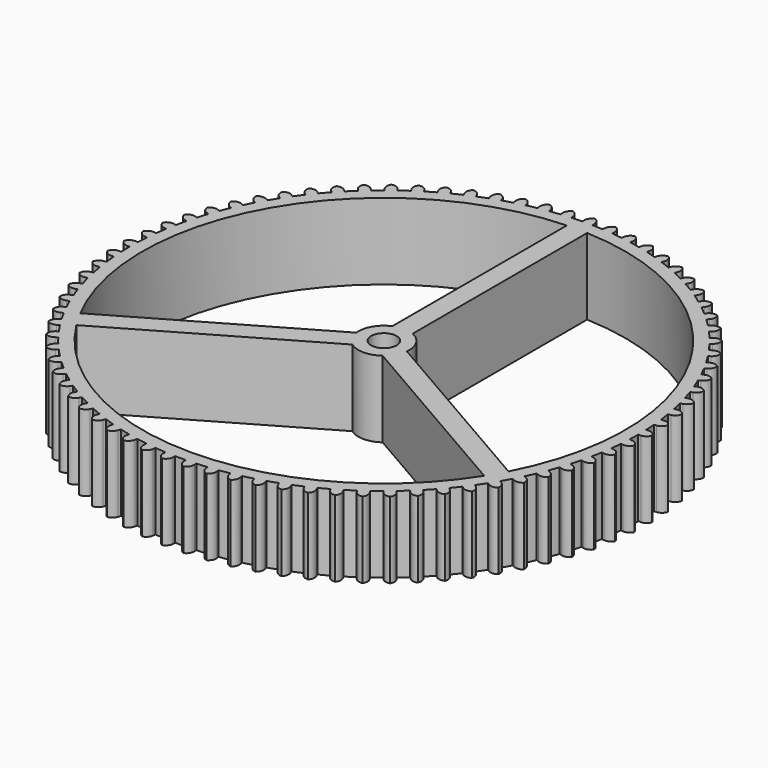
from build123d import *

# Parameters (mm, degrees)
F0_R        = 2.5
F1_DEPTH    = 15
F2_T1_DEPTH = 22.5


# Not quite as in the source:
# - a fillet or chamfer that OpenCascade refuses, or shapes differently, is made with other operations: its cross-section is extruded or revolved along the edge and cut away or added


with BuildPart() as f1:
    # F0 (on Top) → F1 (new body)
    with BuildSketch(Plane.XY):
        with BuildLine():
            Line((-1, 51.9899989998), (-1, 49.9899989998))
            ThreePointArc((-1, 49.9899989998), (-2.0393428715, 49.9583934955), (-3.0778037415, 49.9051813355))
            Line((-3.0778037415, 49.9051813355), (-3.2408225906, 51.8985299491))
            Line((-3.2408225906, 51.8985299491), (-5.2341677556, 51.735511382))
            Line((-5.2341677556, 51.735511382), (-5.0711491885, 49.742166217))
            Line((-5.0711491885, 49.742166217), (-7.1351257823, 49.4882704822))
            Line((-7.1351257823, 49.4882704822), (-7.460078617, 51.4616988431))
            Line((-7.460078617, 51.4616988431), (-9.4335035638, 51.1367465706))
            Line((-9.4335035638, 51.1367465706), (-9.1085512913, 49.1633216238))
            ThreePointArc((-9.1085512913, 49.1633216238), (-10.1289488194, 48.9632681136), (-11.1449653139, 48.7420374527))
            Line((-11.1449653139, 48.7420374527), (-11.6296896267, 50.6824127208))
            Line((-11.6296896267, 50.6824127208), (-13.5700615378, 50.1976892466))
            Line((-13.5700615378, 50.1976892466), (-13.0853380636, 48.2573173355))
            ThreePointArc((-13.0853380636, 48.2573173355), (-14.0860340848, 47.9747576153), (-15.0806375156, 47.6714483047))
            Line((-15.0806375156, 47.6714483047), (-15.7219075461, 49.5658576027))
            Line((-15.7219075461, 49.5658576027), (-17.6163135667, 48.9245886816))
            Line((-17.6163135667, 48.9245886816), (-16.9750446456, 47.030182661))
            ThreePointArc((-16.9750446456, 47.030182661), (-17.949379693, 46.6669971193), (-18.9159511383, 46.2836276323))
            Line((-18.9159511383, 46.2836276323), (-19.7094993403, 48.1194639789))
            Line((-19.7094993403, 48.1194639789), (-21.5453325108, 47.3259171498))
            Line((-21.5453325108, 47.3259171498), (-20.7517856817, 45.4900839793))
            ThreePointArc((-20.7517856817, 45.4900839793), (-21.6932757163, 45.0486895558), (-22.6253828026, 44.5878111532))
            Line((-22.6253828026, 44.5878111532), (-23.5659282438, 46.3528573604))
            Line((-23.5659282438, 46.3528573604), (-25.3309713973, 45.4123135464))
            Line((-25.3309713973, 45.4123135464), (-24.3904275833, 43.6472703928))
            ThreePointArc((-24.3904275833, 43.6472703928), (-25.2928071443, 43.1306044947), (-26.1842468528, 42.5952842462))
            Line((-26.1842468528, 42.5952842462), (-27.2655303584, 44.2777942227))
            Line((-27.2655303584, 44.2777942227), (-28.948037424, 43.1965125878))
            Line((-28.948037424, 43.1965125878), (-27.8667557891, 41.5140055221))
            ThreePointArc((-27.8667557891, 41.5140055221), (-28.7240196893, 40.9255064756), (-29.5688596358, 40.3193068491))
            Line((-29.5688596358, 40.3193068491), (-30.7836854425, 41.9080837686))
            Line((-30.7836854425, 41.9080837686), (-32.3724596133, 40.6932600636))
            Line((-32.3724596133, 40.6932600636), (-31.1576359083, 39.1044858928))
            ThreePointArc((-31.1576359083, 39.1044858928), (-31.964079198, 38.448070062), (-32.756697112, 37.775025216))
            Line((-32.756697112, 37.775025216), (-34.0969807544, 39.2594960302))
            Line((-34.0969807544, 39.2594960302), (-35.5814490004, 37.9192147066))
            Line((-35.5814490004, 37.9192147066), (-34.2411676768, 36.4347464606))
            ThreePointArc((-34.2411676768, 36.4347464606), (-34.9914236088, 35.7147821845), (-35.7265447489, 34.9793711214))
            Line((-35.7265447489, 34.9793711214), (-37.1833668606, 36.349656922))
            Line((-37.1833668606, 36.349656922), (-38.5536502905, 34.8928373307))
            Line((-38.5536502905, 34.8928373307), (-37.0968306992, 33.5225539008))
            ThreePointArc((-37.0968306992, 33.5225539008), (-37.7859064443, 32.743832423), (-38.4586387005, 31.9509491821))
            Line((-38.4586387005, 31.9509491821), (-40.0223043707, 33.1979309432))
            Line((-40.0223043707, 33.1979309432), (-41.2692839744, 31.6342679782))
            Line((-41.2692839744, 31.6342679782), (-39.7056210095, 30.3872883745))
            ThreePointArc((-39.7056210095, 30.3872883745), (-40.3289308821, 29.5549919579), (-40.9347973323, 28.7099130463))
            Line((-40.9347973323, 28.7099130463), (-42.5949006239, 29.82529231))
            Line((-42.5949006239, 29.82529231), (-43.7102779579, 28.1651918905))
            Line((-43.7102779579, 28.1651918905), (-42.0501775384, 27.0498145565))
            Line((-42.0501775384, 27.0498145565), (-43.1385422172, 25.2778312749))
            Line((-43.1385422172, 25.2778312749), (-44.8840354167, 26.2541853762))
            Line((-44.8840354167, 26.2541853762), (-45.8603878288, 24.5086951965))
            Line((-45.8603878288, 24.5086951965), (-44.1148976491, 23.5323427844))
            ThreePointArc((-44.1148976491, 23.5323427844), (-44.5946969692, 22.6098325488), (-45.0552077964, 21.6775438058))
            Line((-45.0552077964, 21.6775438058), (-46.8744749346, 22.5083752692))
            Line((-46.8744749346, 22.5083752692), (-47.7053049606, 20.6891112785))
            Line((-47.7053049606, 20.6891112785), (-45.8860409699, 19.8582812525))
            ThreePointArc((-45.8860409699, 19.8582812525), (-46.289050649, 18.8997324948), (-46.672038977, 17.9330099581))
            Line((-46.672038977, 17.9330099581), (-48.5529731311, 18.6127897373))
            Line((-48.5529731311, 18.6127897373), (-49.2327517343, 16.7318588373))
            Line((-49.2327517343, 16.7318588373), (-47.3518208343, 16.0520802341))
            ThreePointArc((-47.3518208343, 16.0520802341), (-47.6753589094, 15.0638719381), (-47.9782760139, 14.0691489867))
            Line((-47.9782760139, 14.0691489867), (-49.9083598777, 14.5933532595))
            Line((-49.9083598777, 14.5933532595), (-50.4325632435, 12.663272735))
            Line((-50.4325632435, 12.663272735), (-48.502482719, 12.1390693691))
            ThreePointArc((-48.502482719, 12.1390693691), (-48.7443960977, 11.127777898), (-48.9652261154, 10.1116742489))
            Line((-48.9652261154, 10.1116742489), (-50.931615299, 10.4768145223))
            Line((-50.931615299, 10.4768145223), (-51.2967549407, 8.5104287407))
            Line((-51.2967549407, 8.5104287407), (-49.3303691591, 8.1452890991))
            ThreePointArc((-49.3303691591, 8.1452890991), (-49.4890479477, 7.1176444307), (-49.6263212914, 6.0869220862))
            Line((-49.6263212914, 6.0869220862), (-51.6159297993, 6.2905684119))
            Line((-51.6159297993, 6.2905684119), (-51.8195757727, 4.3009633462))
            Line((-51.8195757727, 4.3009633462), (-49.8299707069, 4.0973173728))
            ThreePointArc((-49.8299707069, 4.0973173728), (-49.9043589243, 3.060158313), (-49.9571620624, 2.0216765601))
            Line((-49.9571620624, 2.0216765601), (-51.9567493782, 2.0624737055))
            Line((-51.9567493782, 2.0624737055), (-51.997546453, 0.0628898491))
            Line((-51.997546453, 0.0628898491), (-49.9979625966, 0.0220927743))
            ThreePointArc((-49.9979625966, 0.0220927743), (-49.9875652014, -1.0176785546), (-49.9555467378, -2.057008791))
            Line((-49.9555467378, -2.057008791), (-51.9518059378, -2.1793323243))
            Line((-51.9518059378, -2.1793323243), (-51.8294826162, -4.1755880707))
            Line((-51.8294826162, -4.1755880707), (-49.8332268698, -4.053264749))
            ThreePointArc((-49.8332268698, -4.053264749), (-49.738113055, -5.0887288404), (-49.6214860672, -6.1219909892))
            Line((-49.6214860672, -6.1219909892), (-51.6011323759, -6.4066211582))
            Line((-51.6011323759, -6.4066211582), (-51.3165026994, -8.3862640419))
            Line((-51.3165026994, -8.3862640419), (-49.3368598156, -8.1016343654))
            ThreePointArc((-49.3368598156, -8.1016343654), (-49.157662548, -9.1259003765), (-48.9572031694, -10.1462182485))
            Line((-48.9572031694, -10.1462182485), (-50.9070623672, -10.5912608864))
            Line((-50.9070623672, -10.5912608864), (-50.4620204993, -12.5411167107))
            Line((-50.4620204993, -12.5411167107), (-48.5121646749, -12.0960748428))
            ThreePointArc((-48.5121646749, -12.0960748428), (-48.2500764826, -13.1023264524), (-47.9671187374, -14.1029100005))
            Line((-47.9671187374, -14.1029100005), (-49.874214833, -14.705403422))
            Line((-49.874214833, -14.705403422), (-49.2717224539, -16.6124962181))
            Line((-49.2717224539, -16.6124962181), (-47.3646296577, -16.010003839))
            ThreePointArc((-47.3646296577, -16.010003839), (-47.0213946945, -16.9915446086), (-46.6578216197, -17.9657351144))
            Line((-46.6578216197, -17.9657351144), (-48.5094632032, -18.7216698251))
            Line((-48.5094632032, -18.7216698251), (-47.7535298004, -20.5733082052))
            Line((-47.7535298004, -20.5733082052), (-45.9018914203, -19.8173748023))
            ThreePointArc((-45.9018914203, -19.8173748023), (-45.4797938583, -20.76767274), (-45.0380249727, -21.7089871264))
            Line((-45.0380249727, -21.7089871264), (-46.8218896749, -22.6133325056))
            Line((-46.8218896749, -22.6133325056), (-45.9175458603, -24.3971941216))
            Line((-45.9175458603, -24.3971941216), (-44.1336842443, -23.492850307))
            ThreePointArc((-44.1336842443, -23.492850307), (-43.635533073, -24.4055813369), (-43.1185082758, -25.307755312))
            Line((-43.1185082758, -25.307755312), (-44.8227247714, -26.3544930903))
            Line((-44.8227247714, -26.3544930903), (-43.775988804, -28.0587066375))
            Line((-43.775988804, -28.0587066375), (-42.0717752568, -27.0119706701))
            ThreePointArc((-42.0717752568, -27.0119706701), (-41.5008855901, -27.8810607177), (-40.9120455958, -28.7380904625))
            Line((-40.9120455958, -28.7380904625), (-42.5252726053, -29.9202547728))
            Line((-42.5252726053, -29.9202547728), (-41.3431103402, -31.5334789913))
            Line((-41.3431103402, -31.5334789913), (-39.7298861218, -30.3513167262))
            ThreePointArc((-39.7298861218, -30.3513167262), (-39.0900571362, -31.1709821406), (-38.433320578, -31.9771642636))
            Line((-38.433320578, -31.9771642636), (-39.9448223417, -33.2868879974))
            Line((-39.9448223417, -33.2868879974), (-38.6351008738, -34.7983871461))
            Line((-38.6351008738, -34.7983871461), (-37.1236017251, -33.4886656782))
            ThreePointArc((-37.1236017251, -33.4886656782), (-36.419091377, -34.2534517214), (-35.6988287283, -35.0034212135))
            Line((-35.6988287283, -35.0034212135), (-37.0985464514, -36.4319883755))
            Line((-37.0985464514, -36.4319883755), (-35.6699817609, -37.831703677))
            Line((-35.6699817609, -37.831703677), (-34.2702664594, -36.4031389866))
            ThreePointArc((-34.2702664594, -36.4031389866), (-33.505763149, -37.1079561335), (-32.7267676388, -37.7967220716))
            Line((-32.7267676388, -37.7967220716), (-34.0053864308, -39.3346257829))
            Line((-34.0053864308, -39.3346257829), (-32.4674853801, -40.6132423628))
            Line((-32.4674853801, -40.6132423628), (-31.1888688002, -39.0753413121))
            ThreePointArc((-31.1888688002, -39.0753413121), (-30.3694601708, -39.7154991211), (-29.5369158858, -40.3384778814))
            Line((-29.5369158858, -40.3384778814), (-30.6859267495, -41.9754836467))
            Line((-30.6859267495, -41.9754836467), (-29.0489238163, -43.1244925225))
            Line((-29.0489238163, -43.1244925225), (-27.8999149405, -41.4874895894))
            ThreePointArc((-27.8999149405, -41.4874895894), (-27.0310540213, -42.0587279157), (-26.1505014063, -42.6117736774))
            Line((-26.1505014063, -42.6117736774), (-27.1622578641, -44.3369874933))
            Line((-27.1622578641, -44.3369874933), (-25.4370470329, -45.3487422007))
            Line((-25.4370470329, -45.3487422007), (-24.4252923255, -43.6235313695))
            ThreePointArc((-24.4252923255, -43.6235313695), (-23.5127612426, -44.1220487164), (-22.59006023, -44.6014810512))
            Line((-22.59006023, -44.6014810512), (-23.4578292095, -46.4034219044))
            Line((-23.4578292095, -46.4034219044), (-21.6558914737, -47.2711893827))
            Line((-21.6558914737, -47.2711893827), (-20.7881239955, -45.4692516469))
            ThreePointArc((-20.7881239955, -45.4692516469), (-19.8379954928, -45.8917304637), (-18.8792865055, -46.2943588284))
            Line((-18.8792865055, -46.2943588284), (-19.5972931474, -48.1610350999))
            Line((-19.5972931474, -48.1610350999), (-17.7306201053, -48.8790404996))
            Line((-17.7306201053, -48.8790404996), (-17.0126147056, -47.0123674576))
            ThreePointArc((-17.0126147056, -47.0123674576), (-16.0312117314, -47.3559962174), (-15.0428748197, -47.6791411868))
            Line((-15.0428748197, -47.6791411868), (-15.6063409082, -49.598130454))
            Line((-15.6063409082, -49.598130454), (-13.687354961, -50.1615955677))
            Line((-13.687354961, -50.1615955677), (-13.1238898473, -48.2426096204))
            ThreePointArc((-13.1238898473, -48.2426096204), (-12.1177434765, -48.5051015306), (-11.1063558594, -48.7466126282))
            Line((-11.1063558594, -48.7466126282), (-11.5115316207, -50.7051443341))
            Line((-11.5115316207, -50.7051443341), (-9.5530033032, -51.1103193944))
            Line((-9.5530033032, -51.1103193944), (-9.1478282429, -49.1517910769))
            ThreePointArc((-9.1478282429, -49.1517910769), (-8.1236342136, -49.3313992971), (-7.0959265088, -49.4896693063))
            Line((-7.0959265088, -49.4896693063), (-7.340115565, -51.4747097456))
            Line((-7.340115565, -51.4747097456), (-5.35507856, -51.7188983793))
            Line((-5.35507856, -51.7188983793), (-5.1108899263, -49.7338613743))
            ThreePointArc((-5.1108899263, -49.7338613743), (-4.0754640808, -49.8293906415), (-3.0382755136, -49.9033663016))
            Line((-3.0382755136, -49.9033663016), (-3.1198528268, -51.9017053575))
            Line((-3.1198528268, -51.9017053575), (-1.1215172281, -51.9832825297))
            Line((-1.1215172281, -51.9832825297), (-1.039940056, -49.984946931))
            ThreePointArc((-1.039940056, -49.984946931), (-0.0001729825, -49.9957615135), (1.0395941284, -49.9849505287))
            Line((1.0395941284, -49.9849505287), (1.1211714417, -51.9832895847))
            Line((1.1211714417, -51.9832895847), (3.1195070404, -51.9017124126))
            Line((3.1195070404, -51.9017124126), (3.0379298682, -49.9033768139))
            ThreePointArc((3.0379298682, -49.9033768139), (4.0751186914, -49.8294047425), (5.1105448674, -49.7338790582))
            Line((5.1105448674, -49.7338790582), (5.3547339237, -51.7189194974))
            Line((5.3547339237, -51.7189194974), (7.3397709286, -51.4747308636))
            Line((7.3397709286, -51.4747308636), (7.0955822949, -49.4896938587))
            ThreePointArc((7.0955822949, -49.4896938587), (8.1232905473, -49.3314274054), (9.147485198, -49.1518227291))
            Line((9.147485198, -49.1518227291), (9.5526609593, -51.110354435))
            Line((9.5526609593, -51.110354435), (11.5111892768, -50.7051793747))
            Line((11.5111892768, -50.7051793747), (11.1060142165, -48.7466510572))
            ThreePointArc((11.1060142165, -48.7466510572), (12.1174026693, -48.5051434592), (13.1235499484, -48.2426550304))
            Line((13.1235499484, -48.2426550304), (13.6870160369, -50.1616442976))
            Line((13.6870160369, -50.1616442976), (15.6060019841, -49.5981791839))
            Line((15.6060019841, -49.5981791839), (15.0425368704, -47.6791932367))
            ThreePointArc((15.0425368704, -47.6791932367), (16.0308749003, -47.3560516871), (17.0122790635, -47.0124263231))
            Line((17.0122790635, -47.0124263231), (17.7302857054, -48.8791025946))
            Line((17.7302857054, -48.8791025946), (19.5969587474, -48.1610971949))
            Line((19.5969587474, -48.1610971949), (18.8789533477, -46.2944241528))
            ThreePointArc((18.8789533477, -46.2944241528), (19.8376637281, -45.8917991054), (20.7877936927, -45.4693235762))
            Line((20.7877936927, -45.4693235762), (21.6555626722, -47.2712644295))
            Line((21.6555626722, -47.2712644295), (23.457500408, -46.4034969512))
            Line((23.457500408, -46.4034969512), (22.5897329298, -44.6015592154))
            ThreePointArc((22.5897329298, -44.6015592154), (23.5124356014, -44.1221300734), (24.4249684091, -43.6236158839))
            Line((24.4249684091, -43.6236158839), (25.4367248669, -45.3488296999))
            Line((25.4367248669, -45.3488296999), (27.1619356981, -44.3370749925))
            Line((27.1619356981, -44.3370749925), (26.1501809908, -42.6118641613))
            ThreePointArc((26.1501809908, -42.6118641613), (27.0307355194, -42.0588214465), (27.8995984151, -41.4875861265))
            Line((27.8995984151, -41.4875861265), (29.0486092789, -43.1245918918))
            Line((29.0486092789, -43.1245918918), (30.685612212, -41.9755830159))
            Line((30.685612212, -41.9755830159), (29.5366033361, -40.3385800828))
            ThreePointArc((29.5366033361, -40.3385800828), (30.3691497768, -39.7156042032), (31.1885606212, -39.0754492295))
            Line((31.1885606212, -39.0754492295), (32.4671794132, -40.6133529409))
            Line((32.4671794132, -40.6133529409), (34.0050804639, -39.334736361))
            Line((34.0050804639, -39.334736361), (32.726463884, -37.7968353103))
            ThreePointArc((32.726463884, -37.7968353103), (33.5054617774, -37.1080720677), (34.2699675266, -36.4032575661))
            Line((34.2699675266, -36.4032575661), (35.6696852497, -37.831824728))
            Line((35.6696852497, -37.831824728), (37.0982499402, -36.4321094265))
            Line((37.0982499402, -36.4321094265), (35.6985346387, -35.0035447361))
            ThreePointArc((35.6985346387, -35.0035447361), (36.4187998824, -34.2535777362), (37.1233128768, -33.4887941307))
            Line((37.1233128768, -33.4887941307), (38.6348146405, -34.7985178645))
            Line((38.6348146405, -34.7985178645), (39.9445361084, -33.2870187158))
            Line((39.9445361084, -33.2870187158), (38.4330369597, -31.9772972479))
            ThreePointArc((38.4330369597, -31.9772972479), (39.0897763074, -31.1711173973), (39.7296081291, -30.3514541968))
            Line((39.7296081291, -30.3514541968), (41.3428351386, -31.5336185071))
            Line((41.3428351386, -31.5336185071), (42.5249974036, -29.9203942886))
            Line((42.5249974036, -29.9203942886), (40.9117731851, -28.7382320236))
            ThreePointArc((40.9117731851, -28.7382320236), (41.5006161448, -27.8812043162), (42.0715088187, -27.012116244))
            Line((42.0715088187, -27.012116244), (43.7757253143, -28.0588540224))
            Line((43.7757253143, -28.0588540224), (44.8224612817, -26.3546404751))
            Line((44.8224612817, -26.3546404751), (43.1182477345, -25.3079045077))
            ThreePointArc((43.1182477345, -25.3079045077), (43.6352756534, -24.4057323216), (44.1334299829, -23.4930030154))
            Line((44.1334299829, -23.4930030154), (45.9172946851, -24.3973483946))
            Line((45.9172946851, -24.3973483946), (46.8216384997, -22.6134867786))
            Line((46.8216384997, -22.6134867786), (45.0377768837, -21.709142964))
            ThreePointArc((45.0377768837, -21.709142964), (45.4795490263, -20.7678301062), (45.9016498766, -19.817533629))
            Line((45.9016498766, -19.817533629), (47.7532914601, -20.5734683397))
            Line((47.7532914601, -20.5734683397), (48.5092248629, -18.7218299596))
            Line((48.5092248629, -18.7218299596), (46.6575864829, -17.9658965568))
            ThreePointArc((46.6575864829, -17.9658965568), (47.0211629285, -16.991707309), (47.364401288, -16.010167727))
            Line((47.364401288, -16.010167727), (49.2714973836, -16.6126611485))
            Line((49.2714973836, -16.6126611485), (49.8739897626, -14.7055683523))
            Line((49.8739897626, -14.7055683523), (47.9668969665, -14.1030759732))
            ThreePointArc((47.9668969665, -14.1030759732), (48.2498581739, -13.1024934042), (48.5119498479, -12.0962427015))
            Line((48.5119498479, -12.0962427015), (50.4618090457, -12.5412853394))
            Line((50.4618090457, -12.5412853394), (50.9068509136, -10.591429515))
            Line((50.9068509136, -10.591429515), (48.9569950892, -10.1463876471))
            ThreePointArc((48.9569950892, -10.1463876471), (49.1574579982, -9.1260704687), (49.33665881, -8.1018050776))
            Line((49.33665881, -8.1018050776), (51.3163051187, -8.3864352466))
            Line((51.3163051187, -8.3864352466), (51.6009347952, -6.4067923628))
            Line((51.6009347952, -6.4067923628), (49.6212919114, -6.1221626863))
            ThreePointArc((49.6212919114, -6.1221626863), (49.7379224744, -5.0889009411), (49.8330398721, -4.0534371788))
            Line((49.8330398721, -4.0534371788), (51.8292990721, -4.1757607121))
            Line((51.8292990721, -4.1757607121), (51.9516223938, -2.1795049657))
            Line((51.9516223938, -2.1795049657), (49.9553666474, -2.057181644))
            ThreePointArc((49.9553666474, -2.057181644), (49.9873887073, -1.0178515184), (49.9977897002, 0.0219197745))
            Line((49.9977897002, 0.0219197745), (51.997377016, 0.0627169199))
            Line((51.997377016, 0.0627169199), (51.9565799412, 2.0623007763))
            Line((51.9565799412, 2.0623007763), (49.9569960849, 2.0215037015))
            ThreePointArc((49.9569960849, 2.0215037015), (49.90419654, 3.059985637), (49.8298119114, 4.0971449543))
            Line((49.8298119114, 4.0971449543), (51.8194204193, 4.30079128))
            Line((51.8194204193, 4.30079128), (51.6157744459, 6.2903963457))
            Line((51.6157744459, 6.2903963457), (49.6261693802, 6.0867503723))
            ThreePointArc((49.6261693802, 6.0867503723), (49.4888996029, 7.1174731918), (49.3302243701, 8.1451184092))
            Line((49.3302243701, 8.1451184092), (51.2966135537, 8.5102586826))
            Line((51.2966135537, 8.5102586826), (50.9314739121, 10.4766444642))
            Line((50.9314739121, 10.4766444642), (48.9650881305, 10.1115048225))
            ThreePointArc((48.9650881305, 10.1115048225), (48.7442616285, 11.1276092356), (48.5023517491, 12.1389015438))
            Line((48.5023517491, 12.1389015438), (50.4324356128, 12.6631058166))
            Line((50.4324356128, 12.6631058166), (49.9082322469, 14.5931863411))
            Line((49.9082322469, 14.5931863411), (47.9781517224, 14.0689829752))
            ThreePointArc((47.9781517224, 14.0689829752), (47.6752380597, 15.0637069748), (47.3517034039, 16.0519163903))
            Line((47.3517034039, 16.0519163903), (49.2326375581, 16.7316961695))
            Line((49.2326375581, 16.7316961695), (48.5528589549, 18.6126270695))
            Line((48.5528589549, 18.6126270695), (46.6719280549, 17.9328484664))
            ThreePointArc((46.6719280549, 17.9328484664), (46.2889430719, 18.8995723283), (45.8859367096, 19.8581224804))
            Line((45.8859367096, 19.8581224804), (47.7052038477, 20.6889539438))
            Line((47.7052038477, 20.6889539438), (46.8743738217, 22.5082179345))
            Line((46.8743738217, 22.5082179345), (45.055109831, 21.6773879085))
            ThreePointArc((45.055109831, 21.6773879085), (44.5946022296, 22.609678245), (44.1148061015, 23.5321901407))
            Line((44.1148061015, 23.5321901407), (45.8602993011, 24.508544242))
            Line((45.8602993011, 24.508544242), (44.883946889, 26.2540344217))
            Line((44.883946889, 26.2540344217), (43.1384567093, 25.2776820096))
            ThreePointArc((43.1384567093, 25.2776820096), (42.6034910915, 26.1693345821), (42.0500981618, 27.049669057))
            Line((42.0500981618, 27.049669057), (43.7102014534, 28.1650483207))
            Line((43.7102014534, 28.1650483207), (42.5948241194, 29.8251487402))
            Line((42.5948241194, 29.8251487402), (40.9347236999, 28.7097714062))
            ThreePointArc((40.9347236999, 28.7097714062), (40.3288601738, 29.5548524142), (39.705553181, 30.3871509875))
            Line((39.705553181, 30.3871509875), (41.2692188512, 31.6341327486))
            Line((41.2692188512, 31.6341327486), (40.0222392475, 33.1977957135))
            Line((40.0222392475, 33.1977957135), (38.4585762826, 31.9508161098))
            ThreePointArc((38.4585762826, 31.9508161098), (37.7858467698, 32.7437016785), (37.0967737193, 33.5224255405))
            Line((37.0967737193, 33.5224255405), (38.553595831, 34.8927113412))
            Line((38.553595831, 34.8927113412), (37.1833124011, 36.3495309325))
            Line((37.1833124011, 36.3495309325), (35.7264928098, 34.9792475025))
            ThreePointArc((35.7264928098, 34.9792475025), (34.9913742143, 35.7146611093), (34.2411207735, 36.4346279813))
            Line((34.2411207735, 36.4346279813), (35.5814044159, 37.9190987955))
            Line((35.5814044159, 37.9190987955), (34.0969361699, 39.2593801192))
            Line((34.0969361699, 39.2593801192), (32.7566548462, 37.7749118732))
            ThreePointArc((32.7566548462, 37.7749118732), (31.9640392611, 38.4479594618), (31.1575982427, 39.104378083))
            Line((31.1575982427, 39.104378083), (32.3724240494, 40.6931550025))
            Line((32.3724240494, 40.6931550025), (30.7836498786, 41.9079787075))
            Line((30.7836498786, 41.9079787075), (29.5688261736, 40.3192045366))
            ThreePointArc((29.5688261736, 40.3192045366), (28.7239883247, 40.9254070865), (27.8667264608, 41.5139090992))
            Line((27.8667264608, 41.5139090992), (28.9480099664, 43.1964190757))
            Line((28.9480099664, 43.1964190757), (27.2655029008, 44.2777007106))
            Line((27.2655029008, 44.2777007106), (26.1842212658, 42.595193645))
            ThreePointArc((26.1842212658, 42.595193645), (25.2927834097, 43.130516978), (24.3904056365, 43.6471859985))
            Line((24.3904056365, 43.6471859985), (25.3309510776, 45.4122322057))
            Line((25.3309510776, 45.4122322057), (23.5659079241, 46.3527760197))
            Line((23.5659079241, 46.3527760197), (22.6253641101, 44.5877328661))
            ThreePointArc((22.6253641101, 44.5877328661), (21.6932586185, 45.048614494), (20.7517701112, 45.4900121752))
            Line((20.7517701112, 45.4900121752), (21.5453183132, 47.3258485218))
            Line((21.5453183132, 47.3258485218), (19.7094851427, 48.1193953509))
            Line((19.7094851427, 48.1193953509), (18.9159383136, 46.2835621804))
            ThreePointArc((18.9159383136, 46.2835621804), (17.9493681948, 46.6669350119), (16.9750344041, 47.030123925))
            Line((16.9750344041, 47.030123925), (17.6163044347, 48.924533223))
            Line((17.6163044347, 48.924533223), (15.7218984141, 49.5658021441))
            Line((15.7218984141, 49.5658021441), (15.080629493, 47.6713961235))
            ThreePointArc((15.080629493, 47.6713961235), (14.0860271117, 47.9747088756), (13.0853320682, 48.2572720584))
            Line((13.0853320682, 48.2572720584), (13.570056381, 50.1976473265))
            Line((13.570056381, 50.1976473265), (11.6296844699, 50.6823708007))
            Line((11.6296844699, 50.6823708007), (11.1449609957, 48.7419988895))
            ThreePointArc((11.1449609957, 48.7419988895), (10.1289452667, 48.963233066), (9.1085484308, 49.163290107))
            Line((9.1085484308, 49.163290107), (9.4335012655, 51.1367184679))
            Line((9.4335012655, 51.1367184679), (7.4600763188, 51.4616707404))
            Line((7.4600763188, 51.4616707404), (7.1351240462, 49.4882457936))
            ThreePointArc((7.1351240462, 49.4882457936), (6.1044563866, 49.6259291175), (5.0711483309, 49.7421486701))
            Line((5.0711483309, 49.7421486701), (5.23416718, 51.7354972838))
            Line((5.23416718, 51.7354972838), (3.2408220151, 51.8985158508))
            Line((3.2408220151, 51.8985158508), (3.077803448, 49.9051706859))
            ThreePointArc((3.077803448, 49.9051706859), (2.0393427808, 49.9583868973), (1, 49.9899955397))
            Line((1, 49.9899955397), (1, 51.9899989998))
            Line((1, 51.9899989998), (-1, 51.9899989998))
        make_face()
        with BuildLine():
            Line((-40.0997262765, -25.4609888369), (-2.9686269666, -4.023338655))
            ThreePointArc((-2.9686269666, -4.023338655), (0, -5), (2.9686269666, -4.023338655))
            Line((2.9686269666, -4.023338655), (40.0997262765, -25.4609888369))
            ThreePointArc((40.0997262765, -25.4609888369), (0, -47.5), (-40.0997262765, -25.4609888369))
        make_face(mode=Mode.SUBTRACT)
        Circle(F0_R, mode=Mode.SUBTRACT)
        with BuildLine():
            ThreePointArc((-42.0997262765, -21.9968872218), (-41.1362066798, 23.75), (-2, 47.4578760587))
            Line((-2, 47.4578760587), (-2, 4.582575695))
            ThreePointArc((-2, 4.582575695), (-4.3301270189, 2.5), (-4.9686269666, -0.5592370399))
            Line((-4.9686269666, -0.5592370399), (-42.0997262765, -21.9968872218))
        make_face(mode=Mode.SUBTRACT)
        with BuildLine():
            ThreePointArc((4.9686269666, -0.5592370399), (4.3301270189, 2.5), (2, 4.582575695))
            Line((2, 4.582575695), (2, 47.4578760587))
            ThreePointArc((2, 47.4578760587), (41.1362066798, 23.75), (42.0997262765, -21.9968872218))
            Line((42.0997262765, -21.9968872218), (4.9686269666, -0.5592370399))
        make_face(mode=Mode.SUBTRACT)
    extrude(amount=F1_DEPTH)

    # F2: fillet of radius 1.5 on 154 edges, made by hand

    # F2_s2 → F2_t1 (cut)
    with BuildSketch(Plane.XY.offset(-3.75)):
        with BuildLine():
            ThreePointArc((0.5, 51.9899989998), (-0.5606601718, 51.5506591716), (-1, 50.4899989998))
            Line((-1, 50.4899989998), (-1, 51.9899989998))
            Line((-1, 51.9899989998), (0.5, 51.9899989998))
        make_face()
        with BuildLine():
            ThreePointArc((1, 50.4899989998), (0.5606601718, 51.5506591716), (-0.5, 51.9899989998))
            Line((-0.5, 51.9899989998), (1, 51.9899989998))
            Line((1, 51.9899989998), (1, 50.4899989998))
        make_face()
        with BuildLine():
            ThreePointArc((4.7358308888, 51.7762519255), (3.6428897016, 51.424827615), (3.1185580897, 50.4035069771))
            Line((3.1185580897, 50.4035069771), (3.2408220151, 51.8985158508))
            Line((3.2408220151, 51.8985158508), (4.7358308888, 51.7762519255))
        make_face()
        with BuildLine():
            ThreePointArc((8.9401450289, 51.217956536), (7.8221961695, 50.9567864141), (7.2163621144, 49.9816020303))
            Line((7.2163621144, 49.9816020303), (7.4600763188, 51.4616707404))
            Line((7.4600763188, 51.4616707404), (8.9401450289, 51.217956536))
        make_face()
        with BuildLine():
            ThreePointArc((9.1897870612, 49.6566497578), (8.9286169392, 50.7745986171), (7.9534325555, 51.3804326723))
            Line((7.9534325555, 51.3804326723), (9.4335012655, 51.1367184679))
            Line((9.4335012655, 51.1367184679), (9.1897870612, 49.6566497578))
        make_face()
        with BuildLine():
            ThreePointArc((-3.1185586653, 50.4035210754), (-3.6428902771, 51.4248417133), (-4.7358314643, 51.7762660238))
            Line((-4.7358314643, 51.7762660238), (-3.2408225906, 51.8985299491))
            Line((-3.2408225906, 51.8985299491), (-3.1185586653, 50.4035210754))
        make_face()
        with BuildLine():
            ThreePointArc((-3.7391588818, 51.8577753073), (-4.7604795198, 51.3334436955), (-5.1119038302, 50.2405025083))
            Line((-5.1119038302, 50.2405025083), (-5.2341677556, 51.735511382))
            Line((-5.2341677556, 51.735511382), (-3.7391588818, 51.8577753073))
        make_face()
        with BuildLine():
            ThreePointArc((-7.2163644127, 49.9816301331), (-7.8221984678, 50.9568145168), (-8.9401473271, 51.2179846388))
            Line((-8.9401473271, 51.2179846388), (-7.460078617, 51.4616988431))
            Line((-7.460078617, 51.4616988431), (-7.2163644127, 49.9816301331))
        make_face()
        with BuildLine():
            ThreePointArc((-7.9534348537, 51.380460775), (-8.9286192375, 50.7746267199), (-9.1897893594, 49.6566778605))
            Line((-9.1897893594, 49.6566778605), (-9.4335035638, 51.1367465706))
            Line((-9.4335035638, 51.1367465706), (-7.9534348537, 51.380460775))
        make_face()
        with BuildLine():
            ThreePointArc((-11.266147021, 49.2271337875), (-11.9494517938, 50.1496922258), (-13.08496856, 50.3188701152))
            Line((-13.08496856, 50.3188701152), (-11.6296896267, 50.6824127208))
            Line((-11.6296896267, 50.6824127208), (-11.266147021, 49.2271337875))
        make_face()
        with BuildLine():
            ThreePointArc((-12.1147826045, 50.5612318523), (-13.0373410428, 49.8779270795), (-13.2065189322, 48.7424103133))
            Line((-13.2065189322, 48.7424103133), (-13.5700615378, 50.1976892466))
            Line((-13.5700615378, 50.1976892466), (-12.1147826045, 50.5612318523))
        make_face()
        with BuildLine():
            ThreePointArc((-15.2409558553, 48.1450530873), (-15.9971840651, 49.0088461061), (-17.1427120616, 49.0849059119))
            Line((-17.1427120616, 49.0849059119), (-15.7219075461, 49.5658576027))
            Line((-15.7219075461, 49.5658576027), (-15.2409558553, 48.1450530873))
        make_face()
        with BuildLine():
            ThreePointArc((-16.1955090513, 49.4055403725), (-17.0593020701, 48.6493121626), (-17.1353618759, 47.5037841662))
            Line((-17.1353618759, 47.5037841662), (-17.6163135667, 48.9245886816))
            Line((-17.6163135667, 48.9245886816), (-16.1955090513, 49.4055403725))
        make_face()
        with BuildLine():
            ThreePointArc((-19.1143392184, 46.7425891011), (-19.9384582914, 47.5418683003), (-21.0863742182, 47.5243038571))
            Line((-21.0863742182, 47.5243038571), (-19.7094993403, 48.1194639789))
            Line((-19.7094993403, 48.1194639789), (-19.1143392184, 46.7425891011))
        make_face()
        with BuildLine():
            ThreePointArc((-20.1684576329, 47.9210772717), (-20.9677368321, 47.0969581987), (-20.9501723889, 45.9490422719))
            Line((-20.9501723889, 45.9490422719), (-21.5453325108, 47.3259171498))
            Line((-21.5453325108, 47.3259171498), (-20.1684576329, 47.9210772717))
        make_face()
        with BuildLine():
            ThreePointArc((-22.8605203833, 45.0290749952), (-23.7470459429, 45.7585213036), (-24.8897106089, 45.6474494999))
            Line((-24.8897106089, 45.6474494999), (-23.5659282438, 46.3528573604))
            Line((-23.5659282438, 46.3528573604), (-22.8605203833, 45.0290749952))
        make_face()
        with BuildLine():
            ThreePointArc((-26.4545691322, 43.0159139234), (-27.3976014971, 43.6706729962), (-28.5274106576, 43.4668329965))
            Line((-28.5274106576, 43.4668329965), (-27.2655303584, 44.2777942227))
            Line((-27.2655303584, 44.2777942227), (-26.4545691322, 43.0159139234))
        make_face()
        with BuildLine():
            ThreePointArc((-27.6861571248, 44.0074738139), (-28.3409161976, 43.064441449), (-28.1370761978, 41.9346322885))
            Line((-28.1370761978, 41.9346322885), (-28.948037424, 43.1965125878))
            Line((-28.948037424, 43.1965125878), (-27.6861571248, 44.0074738139))
        make_face()
        with BuildLine():
            ThreePointArc((-24.0071890321, 46.1177214069), (-24.7366353405, 45.2311958473), (-24.6255635368, 44.0885311812))
            Line((-24.6255635368, 44.0885311812), (-25.3309713973, 45.4123135464))
            Line((-25.3309713973, 45.4123135464), (-24.0071890321, 46.1177214069))
        make_face()
        with BuildLine():
            ThreePointArc((-31.1808789852, 41.6043778423), (-31.7565935087, 40.6111143969), (-31.4613418346, 39.5016794355))
            Line((-31.4613418346, 39.5016794355), (-32.3724596133, 40.6932600636))
            Line((-32.3724596133, 40.6932600636), (-31.1808789852, 41.6043778423))
        make_face()
        with BuildLine():
            ThreePointArc((-29.8725676638, 40.7165031405), (-30.8658311092, 41.292217664), (-31.9752660706, 40.9969659899))
            Line((-31.9752660706, 40.9969659899), (-30.7836854425, 41.9080837686))
            Line((-30.7836854425, 41.9080837686), (-29.8725676638, 40.7165031405))
        make_face()
        with BuildLine():
            ThreePointArc((-33.0917697617, 38.1461448457), (-34.1286542833, 38.6389835349), (-35.2103319389, 38.2542850375))
            Line((-35.2103319389, 38.2542850375), (-34.0969807544, 39.2594960302))
            Line((-34.0969807544, 39.2594960302), (-33.0917697617, 38.1461448457))
        make_face()
        with BuildLine():
            ThreePointArc((-34.4680978159, 38.9244256993), (-34.9609365051, 37.8875411777), (-34.5762380077, 36.8058635221))
            Line((-34.5762380077, 36.8058635221), (-35.5814490004, 37.9192147066))
            Line((-35.5814490004, 37.9192147066), (-34.4680978159, 38.9244256993))
        make_face()
        with BuildLine():
            ThreePointArc((-36.0907521671, 35.3219443496), (-37.1643574695, 35.7286274442), (-38.2110794331, 35.2570422285))
            Line((-38.2110794331, 35.2570422285), (-37.1833668606, 36.349656922))
            Line((-37.1833668606, 36.349656922), (-36.0907521671, 35.3219443496))
        make_face()
        with BuildLine():
            ThreePointArc((-37.5259377181, 35.9854520242), (-37.9326208127, 34.9118467219), (-37.4610355971, 33.8651247583))
            Line((-37.4610355971, 33.8651247583), (-38.5536502905, 34.8928373307))
            Line((-38.5536502905, 34.8928373307), (-37.5259377181, 35.9854520242))
        make_face()
        with BuildLine():
            ThreePointArc((-38.849557147, 32.2626962404), (-39.9527385639, 32.5805173315), (-40.9575390735, 32.0251837195))
            Line((-40.9575390735, 32.0251837195), (-40.0223043707, 33.1979309432))
            Line((-40.0223043707, 33.1979309432), (-38.849557147, 32.2626962404))
        make_face()
        with BuildLine():
            ThreePointArc((-40.3340492716, 32.8070152019), (-40.6518703627, 31.703833785), (-40.0965367507, 30.6990332754))
            Line((-40.0965367507, 30.6990332754), (-41.2692839744, 31.6342679782))
            Line((-41.2692839744, 31.6342679782), (-40.3340492716, 32.8070152019))
        make_face()
        with BuildLine():
            ThreePointArc((-41.3498253093, 28.9887593095), (-42.4752413505, 29.2156033503), (-43.4314336244, 28.5802169954))
            Line((-43.4314336244, 28.5802169954), (-42.5949006239, 29.82529231))
            Line((-42.5949006239, 29.82529231), (-41.3498253093, 28.9887593095))
        make_face()
        with BuildLine():
            ThreePointArc((-42.8737449574, 29.4102672051), (-43.1005889982, 28.2848511639), (-42.4652026432, 27.32865889))
            Line((-42.4652026432, 27.32865889), (-43.7102779579, 28.1651918905))
            Line((-43.7102779579, 28.1651918905), (-42.8737449574, 29.4102672051))
        make_face()
        with BuildLine():
            ThreePointArc((-43.5749177819, 25.5219210671), (-44.7150789893, 25.6562784478), (-45.6162997257, 24.9450677414))
            Line((-45.6162997257, 24.9450677414), (-44.8840354167, 26.2541853762))
            Line((-44.8840354167, 26.2541853762), (-43.5749177819, 25.5219210671))
        make_face()
        with BuildLine():
            ThreePointArc((-45.1281235197, 25.8178128313), (-45.2624809004, 24.6776516239), (-44.551270194, 23.7764308874))
            Line((-44.551270194, 23.7764308874), (-45.8603878288, 24.5086951965))
            Line((-45.8603878288, 24.5086951965), (-45.1281235197, 25.8178128313))
        make_face()
        with BuildLine():
            ThreePointArc((-45.5100269416, 21.8852527497), (-46.6573457305, 21.9262293442), (-47.4975974541, 21.1439272762))
            Line((-47.4975974541, 21.1439272762), (-46.8744749346, 22.5083752692))
            Line((-46.8744749346, 22.5083752692), (-45.5100269416, 21.8852527497))
        make_face()
        with BuildLine():
            ThreePointArc((-47.0821824411, 22.0535592716), (-47.1231590356, 20.9062404827), (-46.3408569676, 20.065988759))
            Line((-46.3408569676, 20.065988759), (-47.7053049606, 20.6891112785))
            Line((-47.7053049606, 20.6891112785), (-47.0821824411, 22.0535592716))
        make_face()
        with BuildLine():
            ThreePointArc((-47.1422749561, 18.102955785), (-48.2891161092, 18.0502789007), (-49.0628070835, 17.2020915623))
            Line((-49.0628070835, 17.2020915623), (-48.5529731311, 18.6127897373))
            Line((-48.5529731311, 18.6127897373), (-47.1422749561, 18.102955785))
        make_face()
        with BuildLine():
            ThreePointArc((-48.7229177819, 18.1425570123), (-48.6702408977, 16.9957158592), (-47.8220535593, 16.2220248849))
            Line((-47.8220535593, 16.2220248849), (-49.2327517343, 16.7318588373))
            Line((-49.2327517343, 16.7318588373), (-48.7229177819, 18.1425570123))
        make_face()
        with BuildLine():
            ThreePointArc((-48.4607994843, 14.2002007351), (-49.599530963, 14.0542209281), (-50.3015124021, 13.1457928661))
            Line((-50.3015124021, 13.1457928661), (-49.9083598777, 14.5933532595))
            Line((-49.9083598777, 14.5933532595), (-48.4607994843, 14.2002007351))
        make_face()
        with BuildLine():
            ThreePointArc((-50.0394107191, 14.1108331284), (-49.8934309121, 12.9721016497), (-48.9850028501, 12.2701202106))
            Line((-48.9850028501, 12.2701202106), (-50.4325632435, 12.663272735))
            Line((-50.4325632435, 12.663272735), (-50.0394107191, 14.1108331284))
        make_face()
        with BuildLine():
            ThreePointArc((-49.4568259628, 10.2029597911), (-50.579869697, 9.9646485329), (-51.2054700303, 9.0020251861))
            Line((-51.2054700303, 9.0020251861), (-50.931615299, 10.4768145223))
            Line((-50.931615299, 10.4768145223), (-49.4568259628, 10.2029597911))
        make_face()
        with BuildLine():
            ThreePointArc((-51.0229002095, 9.9852180769), (-50.7845889512, 8.8621743428), (-49.8219656045, 8.2365740095))
            Line((-49.8219656045, 8.2365740095), (-51.2967549407, 8.5104287407))
            Line((-51.2967549407, 8.5104287407), (-51.0229002095, 9.9852180769))
        make_face()
        with BuildLine():
            ThreePointArc((-50.123726, 6.1378339319), (-51.2236083188, 5.8087771446), (-51.7686642793, 4.7983646127))
            Line((-51.7686642793, 4.7983646127), (-51.6159297993, 6.2905684119))
            Line((-51.6159297993, 6.2905684119), (-50.123726, 6.1378339319))
        make_face()
        with BuildLine():
            ThreePointArc((-51.6668412926, 5.7931671455), (-51.3377845053, 4.6932848266), (-50.3273719734, 4.1482288662))
            Line((-50.3273719734, 4.1482288662), (-51.8195757727, 4.3009633462))
            Line((-51.8195757727, 4.3009633462), (-51.6668412926, 5.7931671455))
        make_face()
        with BuildLine():
            ThreePointArc((-50.4570614859, 2.0318758994), (-51.5264628541, 1.6142634016), (-51.9873471843, 0.5627858132))
            Line((-51.9873471843, 0.5627858132), (-51.9567493782, 2.0624737055))
            Line((-51.9567493782, 2.0624737055), (-50.4570614859, 2.0318758994))
        make_face()
        with BuildLine():
            ThreePointArc((-51.9669486469, 1.5625777414), (-51.5493361491, 0.4931763732), (-50.4978585607, 0.032292043))
            Line((-50.4978585607, 0.032292043), (-51.997546453, 0.0628898491))
            Line((-51.997546453, 0.0628898491), (-51.9669486469, 1.5625777414))
        make_face()
        with BuildLine():
            ThreePointArc((-50.4546141281, -2.0875898331), (-51.4864178559, -2.5909788991), (-51.8600634466, -3.6765241341))
            Line((-51.8600634466, -3.6765241341), (-51.9518059378, -2.1793323243))
            Line((-51.9518059378, -2.1793323243), (-50.4546141281, -2.0875898331))
        make_face()
        with BuildLine():
            ThreePointArc((-51.9212251074, -2.6783962609), (-51.4178360414, -3.7101999888), (-50.3322908064, -4.0838455794))
            Line((-50.3322908064, -4.0838455794), (-51.8294826162, -4.1755880707))
            Line((-51.8294826162, -4.1755880707), (-51.9212251074, -2.6783962609))
        make_face()
        with BuildLine():
            ThreePointArc((-50.1164002131, -6.1931489008), (-51.1037398171, -6.7789645638), (-51.3876601185, -7.891353321))
            Line((-51.3876601185, -7.891353321), (-51.6011323759, -6.4066211582))
            Line((-51.6011323759, -6.4066211582), (-50.1164002131, -6.1931489008))
        make_face()
        with BuildLine():
            ThreePointArc((-51.5299749568, -6.9015318791), (-50.9441592937, -7.8888714831), (-49.8317705366, -8.1727917845))
            Line((-49.8317705366, -8.1727917845), (-51.3165026994, -8.3862640419))
            Line((-51.3165026994, -8.3862640419), (-51.5299749568, -6.9015318791))
        make_face()
        with BuildLine():
            ThreePointArc((-49.4446704989, -10.2574794854), (-50.3809753968, -10.9218232389), (-50.5732809662, -12.0536527547))
            Line((-50.5732809662, -12.0536527547), (-50.9070623672, -10.5912608864))
            Line((-50.9070623672, -10.5912608864), (-49.4446704989, -10.2574794854))
        make_face()
        with BuildLine():
            ThreePointArc((-50.7958019002, -11.0787248425), (-50.1314581467, -12.0150297404), (-48.999628631, -12.2073353098))
            Line((-48.999628631, -12.2073353098), (-50.4620204993, -12.5411167107))
            Line((-50.4620204993, -12.5411167107), (-50.7958019002, -11.0787248425))
        make_face()
        with BuildLine():
            ThreePointArc((-48.4438952358, -14.2535341377), (-49.3229344731, -14.9919848835), (-49.4223455487, -16.1357230191))
            Line((-49.4223455487, -16.1357230191), (-49.874214833, -14.705403422))
            Line((-49.874214833, -14.705403422), (-48.4438952358, -14.2535341377))
        make_face()
        with BuildLine():
            ThreePointArc((-49.7235917382, -15.182176621), (-48.9851409923, -16.0612158582), (-47.8414028568, -16.1606269338))
            Line((-47.8414028568, -16.1606269338), (-49.2717224539, -16.6124962181))
            Line((-49.2717224539, -16.6124962181), (-49.7235917382, -15.182176621))
        make_face()
        with BuildLine():
            ThreePointArc((-47.1207344182, -18.154719773), (-47.9366581336, -18.9623632434), (-47.9425131511, -20.1103986102))
            Line((-47.9425131511, -20.1103986102), (-48.5094632032, -18.7216698251))
            Line((-48.5094632032, -18.7216698251), (-47.1207344182, -18.154719773))
        make_face()
        with BuildLine():
            ThreePointArc((-48.3204798525, -19.1845794201), (-47.5128363821, -20.0005031356), (-46.3648010153, -20.006358153))
            Line((-46.3648010153, -20.006358153), (-47.7535298004, -20.5733082052))
            Line((-47.7535298004, -20.5733082052), (-48.3204798525, -19.1845794201))
        make_face()
        with BuildLine():
            ThreePointArc((-45.4839934629, -21.9350746447), (-46.2313718189, -22.8065361055), (-46.143631814, -23.9512287176))
            Line((-46.143631814, -23.9512287176), (-46.8218896749, -22.6133325056))
            Line((-46.8218896749, -22.6133325056), (-45.4839934629, -21.9350746447))
        make_face()
        with BuildLine():
            ThreePointArc((-46.5958037213, -23.0592979096), (-45.7243422604, -23.8066762656), (-44.5796496483, -23.7189362607))
            Line((-44.5796496483, -23.7189362607), (-45.9175458603, -24.3971941216))
            Line((-45.9175458603, -24.3971941216), (-46.5958037213, -23.0592979096))
        make_face()
        with BuildLine():
            ThreePointArc((-43.544564611, -25.5694411148), (-44.2184239278, -26.4989211338), (-44.0376727959, -27.6326532507))
            Line((-44.0376727959, -27.6326532507), (-44.8227247714, -26.3544930903))
            Line((-44.8227247714, -26.3544930903), (-43.544564611, -25.5694411148))
        make_face()
        with BuildLine():
            ThreePointArc((-44.5610407795, -26.7805464771), (-43.6315607605, -27.4544057939), (-42.4978286436, -27.273654662))
            Line((-42.4978286436, -27.273654662), (-43.775988804, -28.0587066375))
            Line((-43.775988804, -28.0587066375), (-44.5610407795, -26.7805464771))
        make_face()
        with BuildLine():
            ThreePointArc((-41.3153544414, -29.033633074), (-41.9112102965, -30.0149461151), (-41.6386509065, -31.1301729367))
            Line((-41.6386509065, -31.1301729367), (-42.5252726053, -29.9202547728))
            Line((-42.5252726053, -29.9202547728), (-41.3153544414, -29.033633074))
        make_face()
        with BuildLine():
            ThreePointArc((-42.229732039, -30.3235608274), (-41.2484189979, -30.9194166825), (-40.1331921764, -30.6468572925))
            Line((-40.1331921764, -30.6468572925), (-41.3431103402, -31.5334789913))
            Line((-41.3431103402, -31.5334789913), (-42.229732039, -30.3235608274))
        make_face()
        with BuildLine():
            ThreePointArc((-38.8111979802, -32.3045968965), (-39.3250850512, -33.3312124832), (-38.9625312408, -34.420512359))
            Line((-38.9625312408, -34.420512359), (-39.9448223417, -33.2868879974))
            Line((-39.9448223417, -33.2868879974), (-38.8111979802, -32.3045968965))
        make_face()
        with BuildLine():
            ThreePointArc((-39.6173919747, -33.6647627846), (-38.590776388, -34.1786498556), (-37.5014765123, -33.8160960452))
            Line((-37.5014765123, -33.8160960452), (-38.6351008738, -34.7983871461))
            Line((-38.6351008738, -34.7983871461), (-39.6173919747, -33.6647627846))
        make_face()
        with BuildLine():
            ThreePointArc((-36.0487599753, -35.3605648577), (-36.4772584285, -36.4256510327), (-36.0271229335, -37.4817748516))
            Line((-36.0271229335, -37.4817748516), (-37.0985464514, -36.4319883755))
            Line((-37.0985464514, -36.4319883755), (-36.0487599753, -35.3605648577))
        make_face()
        with BuildLine():
            ThreePointArc((-36.7414052788, -36.7819172009), (-35.6763191037, -37.2104156541), (-34.6201952848, -36.7602801592))
            Line((-34.6201952848, -36.7602801592), (-35.6699817609, -37.831703677))
            Line((-35.6699817609, -37.831703677), (-36.7414052788, -36.7819172009))
        make_face()
        with BuildLine():
            ThreePointArc((-33.0464239959, -38.1811999949), (-33.3866822448, -39.2776687855), (-32.8519606428, -40.2935882178))
            Line((-32.8519606428, -40.2935882178), (-34.0053864308, -39.3346257829))
            Line((-34.0053864308, -39.3346257829), (-33.0464239959, -38.1811999949))
        make_face()
        with BuildLine():
            ThreePointArc((-33.6209111681, -39.6542799279), (-32.5244423775, -39.9945381768), (-31.5085229452, -39.4598165748))
            Line((-31.5085229452, -39.4598165748), (-32.4674853801, -40.6132423628))
            Line((-32.4674853801, -40.6132423628), (-33.6209111681, -39.6542799279))
        make_face()
        with BuildLine():
            ThreePointArc((-29.8241700926, -40.7477314468), (-30.0739237747, -41.868286034), (-29.4581745496, -42.8372403036))
            Line((-29.4581745496, -42.8372403036), (-30.6859267495, -41.9754836467))
            Line((-30.6859267495, -41.9754836467), (-29.8241700926, -40.7477314468))
        make_face()
        with BuildLine():
            ThreePointArc((-30.2766760162, -42.2627358656), (-29.156121429, -42.5124895477), (-28.1871671594, -41.8967403227))
            Line((-28.1871671594, -41.8967403227), (-29.0489238163, -43.1244925225))
            Line((-29.0489238163, -43.1244925225), (-30.2766760162, -42.2627358656))
        make_face()
        with BuildLine():
            ThreePointArc((-26.4034418335, -43.0430793699), (-26.5610288793, -44.1802626479), (-25.8683497407, -45.0958035239))
            Line((-25.8683497407, -45.0958035239), (-27.1622578641, -44.3369874933))
            Line((-27.1622578641, -44.3369874933), (-26.4034418335, -43.0430793699))
        make_face()
        with BuildLine():
            ThreePointArc((-26.7309551563, -44.5899261702), (-25.5937718783, -44.7475132159), (-24.6782310023, -44.0548340773))
            Line((-24.6782310023, -44.0548340773), (-25.4370470329, -45.3487422007))
            Line((-25.4370470329, -45.3487422007), (-26.7309551563, -44.5899261702))
        make_face()
        with BuildLine():
            ThreePointArc((-22.8070036008, -45.0519686026), (-22.8713752945, -46.1982128042), (-22.1063759077, -47.0542475131))
            Line((-22.1063759077, -47.0542475131), (-23.4578292095, -46.4034219044))
            Line((-23.4578292095, -46.4034219044), (-22.8070036008, -45.0519686026))
        make_face()
        with BuildLine():
            ThreePointArc((-23.0073447756, -46.620363774), (-21.861100574, -46.6847354676), (-21.005065865, -45.9197360808))
            Line((-21.005065865, -45.9197360808), (-21.6558914737, -47.2711893827))
            Line((-21.6558914737, -47.2711893827), (-23.0073447756, -46.620363774))
        make_face()
        with BuildLine():
            ThreePointArc((-19.0587890976, -46.7610303184), (-19.0295170561, -47.9087073776), (-18.1972883658, -48.6995391497))
            Line((-18.1972883658, -48.6995391497), (-19.5972931474, -48.1610350999))
            Line((-19.5972931474, -48.1610350999), (-19.0587890976, -46.7610303184))
        make_face()
        with BuildLine():
            ThreePointArc((-19.1306248869, -48.3405364499), (-17.9829478277, -48.3112644083), (-17.1921160555, -47.4790357181))
            Line((-17.1921160555, -47.4790357181), (-17.7306201053, -48.8790404996))
            Line((-17.7306201053, -48.8790404996), (-19.1306248869, -48.3405364499))
        make_face()
        with BuildLine():
            ThreePointArc((-15.183742073, -48.1588909936), (-15.0610210969, -49.3003633089), (-14.1671014478, -50.0207292892))
            Line((-14.1671014478, -50.0207292892), (-15.6063409082, -49.598130454))
            Line((-15.6063409082, -49.598130454), (-15.183742073, -48.1588909936))
        make_face()
        with BuildLine():
            ThreePointArc((-15.1265944214, -49.7389967324), (-13.9851221061, -49.6162757563), (-13.2647561257, -48.7223561072))
            Line((-13.2647561257, -48.7223561072), (-13.687354961, -50.1615955677))
            Line((-13.687354961, -50.1615955677), (-15.1265944214, -49.7389967324))
        make_face()
        with BuildLine():
            ThreePointArc((-11.2076503255, -49.236248096), (-10.9922971027, -50.3639193575), (-10.0426353825, -51.0090256293))
            Line((-10.0426353825, -51.0090256293), (-11.5115316207, -50.7051443341))
            Line((-11.5115316207, -50.7051443341), (-11.2076503255, -49.236248096))
        make_face()
        with BuildLine():
            ThreePointArc((-11.0218995413, -50.8064380992), (-9.8942282798, -50.5910848764), (-9.2491220079, -49.6414231563))
            Line((-9.2491220079, -49.6414231563), (-9.5530033032, -51.1103193944))
            Line((-9.5530033032, -51.1103193944), (-11.0218995413, -50.8064380992))
        make_face()
        with BuildLine():
            ThreePointArc((-3.0586699477, -50.4029536585), (-2.6629585671, -51.4806511986), (-1.6211011278, -51.9628882366))
            Line((-1.6211011278, -51.9628882366), (-3.1198528268, -51.9017053575))
            Line((-3.1198528268, -51.9017053575), (-3.0586699477, -50.4029536585))
        make_face()
        with BuildLine():
            ThreePointArc((-7.1569740897, -49.9859319918), (-6.8504217604, -51.0922977334), (-5.8513378113, -51.6578512209))
            Line((-5.8513378113, -51.6578512209), (-7.340115565, -51.4747097456))
            Line((-7.340115565, -51.4747097456), (-7.1569740897, -49.9859319918))
        make_face()
        with BuildLine():
            ThreePointArc((-2.6202689272, -51.9220996506), (-1.5425713871, -51.5263882699), (-1.060334349, -50.4845308307))
            Line((-1.060334349, -50.4845308307), (-1.1215172281, -51.9832825297))
            Line((-1.1215172281, -51.9832825297), (-2.6202689272, -51.9220996506))
        make_face()
        with BuildLine():
            ThreePointArc((1.0599885626, -50.4845378857), (1.5422256006, -51.526395325), (2.6199231407, -51.9221067056))
            Line((2.6199231407, -51.9221067056), (1.1211714417, -51.9832895847))
            Line((1.1211714417, -51.9832895847), (1.0599885626, -50.4845378857))
        make_face()
        with BuildLine():
            ThreePointArc((-6.8438563138, -51.535756904), (-5.7374905722, -51.2292045747), (-5.1719370847, -50.2301206256))
            Line((-5.1719370847, -50.2301206256), (-5.35507856, -51.7188983793))
            Line((-5.35507856, -51.7188983793), (-6.8438563138, -51.535756904))
        make_face()
        with BuildLine():
            ThreePointArc((1.6207553413, -51.9628952916), (2.6626127806, -51.4806582536), (3.0583241613, -50.4029607135))
            Line((3.0583241613, -50.4029607135), (3.1195070404, -51.9017124126))
            Line((3.1195070404, -51.9017124126), (1.6207553413, -51.9628952916))
        make_face()
        with BuildLine():
            ThreePointArc((5.1715924483, -50.2301417437), (5.7371459358, -51.2292256928), (6.8435116774, -51.5357780221))
            Line((6.8435116774, -51.5357780221), (5.3547339237, -51.7189194974))
            Line((5.3547339237, -51.7189194974), (5.1715924483, -50.2301417437))
        make_face()
        with BuildLine():
            ThreePointArc((5.8509931749, -51.657872339), (6.850077124, -51.0923188515), (7.1566294533, -49.9859531099))
            Line((7.1566294533, -49.9859531099), (7.3397709286, -51.4747308636))
            Line((7.3397709286, -51.4747308636), (5.8509931749, -51.657872339))
        make_face()
        with BuildLine():
            ThreePointArc((9.2487796641, -49.6414581969), (9.8938859359, -50.591119917), (11.0215571975, -50.8064731398))
            Line((11.0215571975, -50.8064731398), (9.5526609593, -51.110354435))
            Line((9.5526609593, -51.110354435), (9.2487796641, -49.6414581969))
        make_face()
        with BuildLine():
            ThreePointArc((10.0422930387, -51.0090606699), (10.9919547589, -50.3639543981), (11.2073079816, -49.2362831366))
            Line((11.2073079816, -49.2362831366), (11.5111892768, -50.7051793747))
            Line((11.5111892768, -50.7051793747), (10.0422930387, -51.0090606699))
        make_face()
        with BuildLine():
            ThreePointArc((13.2644172016, -48.7224048372), (13.984783182, -49.6163244863), (15.1262554973, -49.7390454623))
            Line((15.1262554973, -49.7390454623), (13.6870160369, -50.1616442976))
            Line((13.6870160369, -50.1616442976), (13.2644172016, -48.7224048372))
        make_face()
        with BuildLine():
            ThreePointArc((14.1667625237, -50.0207780192), (15.0606821728, -49.3004120388), (15.1834031488, -48.1589397235))
            Line((15.1834031488, -48.1589397235), (15.6060019841, -49.5981791839))
            Line((15.6060019841, -49.5981791839), (14.1667625237, -50.0207780192))
        make_face()
        with BuildLine():
            ThreePointArc((17.1917816556, -47.479097813), (17.9826134277, -48.3113265033), (19.1302904869, -48.3405985448))
            Line((19.1302904869, -48.3405985448), (17.7302857054, -48.8791025946))
            Line((17.7302857054, -48.8791025946), (17.1917816556, -47.479097813))
        make_face()
        with BuildLine():
            ThreePointArc((18.1969539659, -48.6996012447), (19.0291826561, -47.9087694726), (19.0584546977, -46.7610924134))
            Line((19.0584546977, -46.7610924134), (19.5969587474, -48.1610971949))
            Line((19.5969587474, -48.1610971949), (18.1969539659, -48.6996012447))
        make_face()
        with BuildLine():
            ThreePointArc((21.0047370636, -45.9198111276), (21.8607717725, -46.6848105144), (23.0070159741, -46.6204388208))
            Line((23.0070159741, -46.6204388208), (21.6555626722, -47.2712644295))
            Line((21.6555626722, -47.2712644295), (21.0047370636, -45.9198111276))
        make_face()
        with BuildLine():
            ThreePointArc((22.1060471062, -47.0543225599), (22.871046493, -46.198287851), (22.8066747994, -45.0520436494))
            Line((22.8066747994, -45.0520436494), (23.457500408, -46.4034969512))
            Line((23.457500408, -46.4034969512), (22.1060471062, -47.0543225599))
        make_face()
        with BuildLine():
            ThreePointArc((24.6779088364, -44.0549215765), (25.5934497124, -44.7476007151), (26.7306329903, -44.5900136694))
            Line((26.7306329903, -44.5900136694), (25.4367248669, -45.3488296999))
            Line((25.4367248669, -45.3488296999), (24.6779088364, -44.0549215765))
        make_face()
        with BuildLine():
            ThreePointArc((25.8680275747, -45.095891023), (26.5607067133, -44.1803501471), (26.4031196676, -43.0431668691))
            Line((26.4031196676, -43.0431668691), (27.1619356981, -44.3370749925))
            Line((27.1619356981, -44.3370749925), (25.8680275747, -45.095891023))
        make_face()
        with BuildLine():
            ThreePointArc((28.186852622, -41.896839692), (29.1558068915, -42.512588917), (30.2763614787, -42.2628352349))
            Line((30.2763614787, -42.2628352349), (29.0486092789, -43.1245918918))
            Line((29.0486092789, -43.1245918918), (28.186852622, -41.896839692))
        make_face()
        with BuildLine():
            ThreePointArc((29.4578600122, -42.8373396729), (30.0736092372, -41.8683854033), (29.8238555551, -40.7478308161))
            Line((29.8238555551, -40.7478308161), (30.685612212, -41.9755830159))
            Line((30.685612212, -41.9755830159), (29.4578600122, -42.8373396729))
        make_face()
        with BuildLine():
            ThreePointArc((31.5082169783, -39.4599271529), (32.5241364106, -39.9946487549), (33.6206052012, -39.654390506))
            Line((33.6206052012, -39.654390506), (32.4671794132, -40.6133529409))
            Line((32.4671794132, -40.6133529409), (31.5082169783, -39.4599271529))
        make_face()
        with BuildLine():
            ThreePointArc((32.8516546759, -40.2936987959), (33.3863762779, -39.2777793636), (33.046118029, -38.181310573))
            Line((33.046118029, -38.181310573), (34.0050804639, -39.334736361))
            Line((34.0050804639, -39.334736361), (32.8516546759, -40.2936987959))
        make_face()
        with BuildLine():
            ThreePointArc((34.6198987736, -36.7604012102), (35.6760225925, -37.2105367051), (36.7411087676, -36.7820382519))
            Line((36.7411087676, -36.7820382519), (35.6696852497, -37.831824728))
            Line((35.6696852497, -37.831824728), (34.6198987736, -36.7604012102))
        make_face()
        with BuildLine():
            ThreePointArc((36.0268264223, -37.4818959026), (36.4769619173, -36.4257720837), (36.0484634641, -35.3606859087))
            Line((36.0484634641, -35.3606859087), (37.0982499402, -36.4321094265))
            Line((37.0982499402, -36.4321094265), (36.0268264223, -37.4818959026))
        make_face()
        with BuildLine():
            ThreePointArc((37.5011902789, -33.8162267636), (38.5904901547, -34.178780574), (39.6171057414, -33.664893503))
            Line((39.6171057414, -33.664893503), (38.6348146405, -34.7985178645))
            Line((38.6348146405, -34.7985178645), (37.5011902789, -33.8162267636))
        make_face()
        with BuildLine():
            ThreePointArc((38.9622450074, -34.4206430773), (39.3247988178, -33.3313432016), (38.8109117468, -32.3047276149))
            Line((38.8109117468, -32.3047276149), (39.9445361084, -33.2870187158))
            Line((39.9445361084, -33.2870187158), (38.9622450074, -34.4206430773))
        make_face()
        with BuildLine():
            ThreePointArc((40.1329169747, -30.6469968083), (41.2481437963, -30.9195561984), (42.2294568373, -30.3237003433))
            Line((42.2294568373, -30.3237003433), (41.3428351386, -31.5336185071))
            Line((41.3428351386, -31.5336185071), (40.1329169747, -30.6469968083))
        make_face()
        with BuildLine():
            ThreePointArc((41.6383757048, -31.1303124525), (41.9109350949, -30.0150856309), (41.3150792398, -29.0337725898))
            Line((41.3150792398, -29.0337725898), (42.5249974036, -29.9203942886))
            Line((42.5249974036, -29.9203942886), (41.6383757048, -31.1303124525))
        make_face()
        with BuildLine():
            ThreePointArc((42.4975651539, -27.2738020468), (43.6312972709, -27.4545531788), (44.5607772899, -26.7806938619))
            Line((44.5607772899, -26.7806938619), (43.7757253143, -28.0588540224))
            Line((43.7757253143, -28.0588540224), (42.4975651539, -27.2738020468))
        make_face()
        with BuildLine():
            ThreePointArc((44.0374093062, -27.6328006355), (44.2181604381, -26.4990685186), (43.5443011213, -25.5695884996))
            Line((43.5443011213, -25.5695884996), (44.8224612817, -26.3546404751))
            Line((44.8224612817, -26.3546404751), (44.0374093062, -27.6328006355))
        make_face()
        with BuildLine():
            ThreePointArc((13.0849634032, 50.318828195), (11.949446637, 50.1496503057), (11.2661418642, 49.2270918673))
            Line((11.2661418642, 49.2270918673), (11.6296844699, 50.6823708007))
            Line((11.6296844699, 50.6823708007), (13.0849634032, 50.318828195))
        make_face()
        with BuildLine():
            ThreePointArc((13.2065137754, 48.7423683931), (13.037335886, 49.8778851594), (12.1147774477, 50.5611899321))
            Line((12.1147774477, 50.5611899321), (13.570056381, 50.1976473265))
            Line((13.570056381, 50.1976473265), (13.2065137754, 48.7423683931))
        make_face()
        with BuildLine():
            ThreePointArc((17.1427029295, 49.0848504533), (15.9971749331, 49.0087906475), (15.2409467232, 48.1449976287))
            Line((15.2409467232, 48.1449976287), (15.7218984141, 49.5658021441))
            Line((15.7218984141, 49.5658021441), (17.1427029295, 49.0848504533))
        make_face()
        with BuildLine():
            ThreePointArc((17.1353527438, 47.5037287076), (17.059292938, 48.649256704), (16.1954999192, 49.4054849138))
            Line((16.1954999192, 49.4054849138), (17.6163044347, 48.924533223))
            Line((17.6163044347, 48.924533223), (17.1353527438, 47.5037287076))
        make_face()
        with BuildLine():
            ThreePointArc((21.0863600206, 47.5242352291), (19.9384440938, 47.5417996723), (19.1143250209, 46.7425204731))
            Line((19.1143250209, 46.7425204731), (19.7094851427, 48.1193953509))
            Line((19.7094851427, 48.1193953509), (21.0863600206, 47.5242352291))
        make_face()
        with BuildLine():
            ThreePointArc((20.9501581914, 45.9489736439), (20.9677226346, 47.0968895707), (20.1684434354, 47.9210086437))
            Line((20.1684434354, 47.9210086437), (21.5453183132, 47.3258485218))
            Line((21.5453183132, 47.3258485218), (20.9501581914, 45.9489736439))
        make_face()
        with BuildLine():
            ThreePointArc((24.8896902893, 45.6473681592), (23.7470256232, 45.7584399629), (22.8605000636, 45.0289936545))
            Line((22.8605000636, 45.0289936545), (23.5659079241, 46.3527760197))
            Line((23.5659079241, 46.3527760197), (24.8896902893, 45.6473681592))
        make_face()
        with BuildLine():
            ThreePointArc((24.6255432172, 44.0884498406), (24.7366150209, 45.2311145066), (24.0071687125, 46.1176400662))
            Line((24.0071687125, 46.1176400662), (25.3309510776, 45.4122322057))
            Line((25.3309510776, 45.4122322057), (24.6255432172, 44.0884498406))
        make_face()
        with BuildLine():
            ThreePointArc((28.5273832, 43.4667394844), (27.3975740395, 43.6705794841), (26.4545416746, 43.0158204114))
            Line((26.4545416746, 43.0158204114), (27.2655029008, 44.2777007106))
            Line((27.2655029008, 44.2777007106), (28.5273832, 43.4667394844))
        make_face()
        with BuildLine():
            ThreePointArc((28.1370487402, 41.9345387765), (28.3408887399, 43.064347937), (27.6861296672, 44.0073803019))
            Line((27.6861296672, 44.0073803019), (28.9480099664, 43.1964190757))
            Line((28.9480099664, 43.1964190757), (28.1370487402, 41.9345387765))
        make_face()
        with BuildLine():
            ThreePointArc((31.9752305067, 40.9968609288), (30.8657955453, 41.2921126029), (29.8725320999, 40.7163980794))
            Line((29.8725320999, 40.7163980794), (30.7836498786, 41.9079787075))
            Line((30.7836498786, 41.9079787075), (31.9752305067, 40.9968609288))
        make_face()
        with BuildLine():
            ThreePointArc((31.4613062707, 39.5015743744), (31.7565579448, 40.6110093358), (31.1808434213, 41.6042727812))
            Line((31.1808434213, 41.6042727812), (32.3724240494, 40.6931550025))
            Line((32.3724240494, 40.6931550025), (31.4613062707, 39.5015743744))
        make_face()
        with BuildLine():
            ThreePointArc((35.2102873544, 38.2541691265), (34.1286096988, 38.6388676239), (33.0917251771, 38.1460289347))
            Line((33.0917251771, 38.1460289347), (34.0969361699, 39.2593801192))
            Line((34.0969361699, 39.2593801192), (35.2102873544, 38.2541691265))
        make_face()
        with BuildLine():
            ThreePointArc((34.5761934232, 36.805747611), (34.9608919206, 37.8874252667), (34.4680532314, 38.9243097883))
            Line((34.4680532314, 38.9243097883), (35.5814044159, 37.9190987955))
            Line((35.5814044159, 37.9190987955), (34.5761934232, 36.805747611))
        make_face()
        with BuildLine():
            ThreePointArc((38.2110249735, 35.256916239), (37.1643030099, 35.7285014546), (36.0906977076, 35.32181836))
            Line((36.0906977076, 35.32181836), (37.1833124011, 36.3495309325))
            Line((37.1833124011, 36.3495309325), (38.2110249735, 35.256916239))
        make_face()
        with BuildLine():
            ThreePointArc((37.4609811375, 33.8649987687), (37.9325663532, 34.9117207323), (37.5258832586, 35.9853260347))
            Line((37.5258832586, 35.9853260347), (38.553595831, 34.8927113412))
            Line((38.553595831, 34.8927113412), (37.4609811375, 33.8649987687))
        make_face()
        with BuildLine():
            ThreePointArc((40.9574739503, 32.0250484898), (39.9526734408, 32.5803821019), (38.8494920238, 32.2625610107))
            Line((38.8494920238, 32.2625610107), (40.0222392475, 33.1977957135))
            Line((40.0222392475, 33.1977957135), (40.9574739503, 32.0250484898))
        make_face()
        with BuildLine():
            ThreePointArc((40.0964716275, 30.6988980458), (40.6518052396, 31.7036985553), (40.3339841484, 32.8068799723))
            Line((40.3339841484, 32.8068799723), (41.2692188512, 31.6341327486))
            Line((41.2692188512, 31.6341327486), (40.0964716275, 30.6988980458))
        make_face()
        with BuildLine():
            ThreePointArc((43.4313571199, 28.5800734256), (42.475164846, 29.2154597805), (41.3497488048, 28.9886157397))
            Line((41.3497488048, 28.9886157397), (42.5948241194, 29.8251487402))
            Line((42.5948241194, 29.8251487402), (43.4313571199, 28.5800734256))
        make_face()
        with BuildLine():
            ThreePointArc((42.4651261388, 27.3285153202), (43.1005124937, 28.2847075941), (42.8736684529, 29.4101236353))
            Line((42.8736684529, 29.4101236353), (43.7102014534, 28.1650483207))
            Line((43.7102014534, 28.1650483207), (42.4651261388, 27.3285153202))
        make_face()
        with BuildLine():
            ThreePointArc((45.616211198, 24.9449167869), (44.7149904616, 25.6561274933), (43.5748292542, 25.5217701126))
            Line((43.5748292542, 25.5217701126), (44.883946889, 26.2540344217))
            Line((44.883946889, 26.2540344217), (45.616211198, 24.9449167869))
        make_face()
        with BuildLine():
            ThreePointArc((44.5511816663, 23.7762799329), (45.2623923727, 24.6775006693), (45.128034992, 25.8176618767))
            Line((45.128034992, 25.8176618767), (45.8602993011, 24.508544242))
            Line((45.8602993011, 24.508544242), (44.5511816663, 23.7762799329))
        make_face()
        with BuildLine():
            ThreePointArc((47.4974963412, 21.1437699415), (46.6572446176, 21.9260720095), (45.5099258287, 21.885095415))
            Line((45.5099258287, 21.885095415), (46.8743738217, 22.5082179345))
            Line((46.8743738217, 22.5082179345), (47.4974963412, 21.1437699415))
        make_face()
        with BuildLine():
            ThreePointArc((46.3407558547, 20.0658314243), (47.1230579227, 20.906083148), (47.0820813282, 22.0534019369))
            Line((47.0820813282, 22.0534019369), (47.7052038477, 20.6889539438))
            Line((47.7052038477, 20.6889539438), (46.3407558547, 20.0658314243))
        make_face()
        with BuildLine():
            ThreePointArc((49.0626929073, 17.2019288945), (48.2890019331, 18.0501162329), (47.1421607799, 18.1027931172))
            Line((47.1421607799, 18.1027931172), (48.5528589549, 18.6126270695))
            Line((48.5528589549, 18.6126270695), (49.0626929073, 17.2019288945))
        make_face()
        with BuildLine():
            ThreePointArc((47.8219393831, 16.2218622171), (48.6701267215, 16.9955531914), (48.7228036057, 18.1423943445))
            Line((48.7228036057, 18.1423943445), (49.2326375581, 16.7316961695))
            Line((49.2326375581, 16.7316961695), (47.8219393831, 16.2218622171))
        make_face()
        with BuildLine():
            ThreePointArc((50.3013847713, 13.1456259477), (49.5994033322, 14.0540540097), (48.4606718535, 14.2000338167))
            Line((48.4606718535, 14.2000338167), (49.9082322469, 14.5931863411))
            Line((49.9082322469, 14.5931863411), (50.3013847713, 13.1456259477))
        make_face()
        with BuildLine():
            ThreePointArc((48.9848752194, 12.2699532922), (49.8933032814, 12.9719347313), (50.0392830884, 14.11066621))
            Line((50.0392830884, 14.11066621), (50.4324356128, 12.6631058166))
            Line((50.4324356128, 12.6631058166), (48.9848752194, 12.2699532922))
        make_face()
        with BuildLine():
            ThreePointArc((51.7685089259, 4.7981925464), (51.2234529655, 5.8086050783), (50.1235706466, 6.1376618657))
            Line((50.1235706466, 6.1376618657), (51.6157744459, 6.2903963457))
            Line((51.6157744459, 6.2903963457), (51.7685089259, 4.7981925464))
        make_face()
        with BuildLine():
            ThreePointArc((50.32721662, 4.1480567999), (51.3376291519, 4.6931127604), (51.6666859392, 5.7929950793))
            Line((51.6666859392, 5.7929950793), (51.8194204193, 4.30079128))
            Line((51.8194204193, 4.30079128), (50.32721662, 4.1480567999))
        make_face()
        with BuildLine():
            ThreePointArc((49.8218242175, 8.2364039513), (50.7844475643, 8.8620042846), (51.0227588225, 9.9850480188))
            Line((51.0227588225, 9.9850480188), (51.2966135537, 8.5102586826))
            Line((51.2966135537, 8.5102586826), (49.8218242175, 8.2364039513))
        make_face()
        with BuildLine():
            ThreePointArc((51.2053286433, 9.001855128), (50.57972831, 9.9644784747), (49.4566845759, 10.2027897329))
            Line((49.4566845759, 10.2027897329), (50.9314739121, 10.4766444642))
            Line((50.9314739121, 10.4766444642), (51.2053286433, 9.001855128))
        make_face()
        with BuildLine():
            ThreePointArc((5.1119032547, 50.24048841), (4.7604789442, 51.3334295972), (3.7391583063, 51.8577612091))
            Line((3.7391583063, 51.8577612091), (5.23416718, 51.7354972838))
            Line((5.23416718, 51.7354972838), (5.1119032547, 50.24048841))
        make_face()
        with BuildLine():
            ThreePointArc((51.9871777473, 0.562612884), (51.5262934172, 1.6140904724), (50.456892049, 2.0317029702))
            Line((50.456892049, 2.0317029702), (51.9565799412, 2.0623007763))
            Line((51.9565799412, 2.0623007763), (51.9871777473, 0.562612884))
        make_face()
        with BuildLine():
            ThreePointArc((50.4976891237, 0.0321191138), (51.5491667121, 0.493003444), (51.9667792099, 1.5624048122))
            Line((51.9667792099, 1.5624048122), (51.997377016, 0.0627169199))
            Line((51.997377016, 0.0627169199), (50.4976891237, 0.0321191138))
        make_face()
        with BuildLine():
            ThreePointArc((51.8598799026, -3.6766967755), (51.4862343119, -2.5911515405), (50.454430584, -2.0877624745))
            Line((50.454430584, -2.0877624745), (51.9516223938, -2.1795049657))
            Line((51.9516223938, -2.1795049657), (51.8598799026, -3.6766967755))
        make_face()
        with BuildLine():
            ThreePointArc((50.3321072624, -4.0840182208), (51.4176524974, -3.7103726302), (51.9210415634, -2.6785689023))
            Line((51.9210415634, -2.6785689023), (51.8292990721, -4.1757607121))
            Line((51.8292990721, -4.1757607121), (50.3321072624, -4.0840182208))
        make_face()
        with BuildLine():
            ThreePointArc((51.3874625378, -7.8915245257), (51.1035422364, -6.7791357685), (50.1162026324, -6.1933201054))
            Line((50.1162026324, -6.1933201054), (51.6009347952, -6.4067923628))
            Line((51.6009347952, -6.4067923628), (51.3874625378, -7.8915245257))
        make_face()
        with BuildLine():
            ThreePointArc((49.8315729558, -8.1729629892), (50.943961713, -7.8890426878), (51.5297773761, -6.9017030838))
            Line((51.5297773761, -6.9017030838), (51.3163051187, -8.3864352466))
            Line((51.3163051187, -8.3864352466), (49.8315729558, -8.1729629892))
        make_face()
        with BuildLine():
            ThreePointArc((50.5730695126, -12.0538213833), (50.3807639432, -10.9219918676), (49.4444590453, -10.2576481141))
            Line((49.4444590453, -10.2576481141), (50.9068509136, -10.591429515))
            Line((50.9068509136, -10.591429515), (50.5730695126, -12.0538213833))
        make_face()
        with BuildLine():
            ThreePointArc((48.9994171774, -12.2075039384), (50.1312466931, -12.015198369), (50.7955904466, -11.0788934711))
            Line((50.7955904466, -11.0788934711), (50.4618090457, -12.5412853394))
            Line((50.4618090457, -12.5412853394), (48.9994171774, -12.2075039384))
        make_face()
        with BuildLine():
            ThreePointArc((49.4221204783, -16.1358879494), (49.3227094027, -14.9921498139), (48.4436701655, -14.253699068))
            Line((48.4436701655, -14.253699068), (49.8739897626, -14.7055683523))
            Line((49.8739897626, -14.7055683523), (49.4221204783, -16.1358879494))
        make_face()
        with BuildLine():
            ThreePointArc((47.8411777865, -16.1607918642), (48.984915922, -16.0613807886), (49.7233666679, -15.1823415514))
            Line((49.7233666679, -15.1823415514), (49.2714973836, -16.6126611485))
            Line((49.2714973836, -16.6126611485), (47.8411777865, -16.1607918642))
        make_face()
        with BuildLine():
            ThreePointArc((47.9422748108, -20.1105587447), (47.9364197933, -18.9625233779), (47.1204960779, -18.1548799075))
            Line((47.1204960779, -18.1548799075), (48.5092248629, -18.7218299596))
            Line((48.5092248629, -18.7218299596), (47.9422748108, -20.1105587447))
        make_face()
        with BuildLine():
            ThreePointArc((46.364562675, -20.0065182875), (47.5125980418, -20.0006632701), (48.3202415122, -19.1847395546))
            Line((48.3202415122, -19.1847395546), (47.7532914601, -20.5734683397))
            Line((47.7532914601, -20.5734683397), (46.364562675, -20.0065182875))
        make_face()
        with BuildLine():
            ThreePointArc((46.1433806388, -23.9513829906), (46.2311206437, -22.8066903785), (45.4837422877, -21.9352289177))
            Line((45.4837422877, -21.9352289177), (46.8216384997, -22.6134867786))
            Line((46.8216384997, -22.6134867786), (46.1433806388, -23.9513829906))
        make_face()
        with BuildLine():
            ThreePointArc((44.5793984731, -23.7190905337), (45.7240910852, -23.8068305385), (46.5955525461, -23.0594521826))
            Line((46.5955525461, -23.0594521826), (45.9172946851, -24.3973483946))
            Line((45.9172946851, -24.3973483946), (44.5793984731, -23.7190905337))
        make_face()
    extrude(amount=F2_T1_DEPTH, mode=Mode.SUBTRACT)


solid = f1.part
